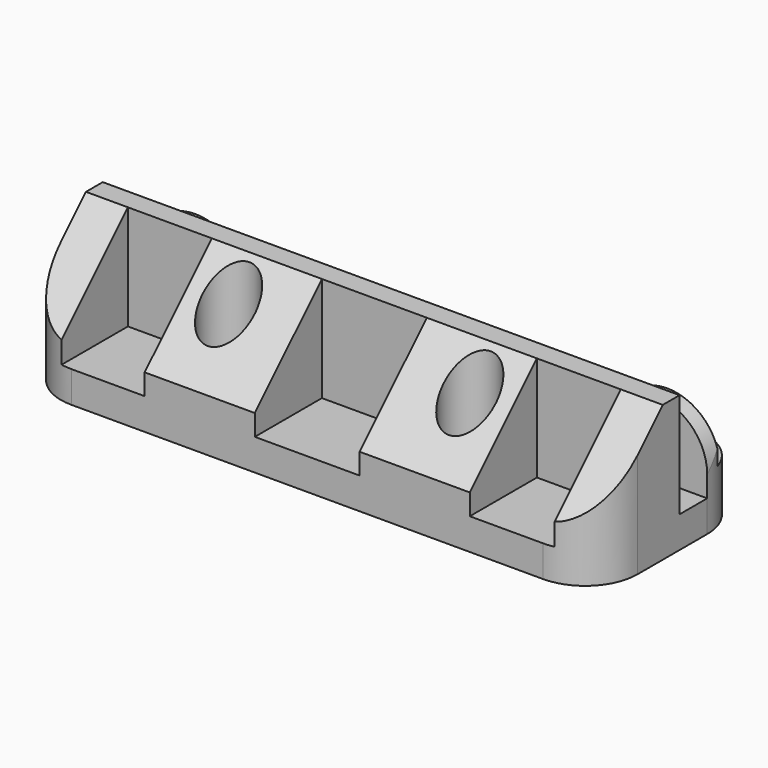
from build123d import *

# Parameters (mm, degrees)
F0_W         = 55
F0_H         = 18.3
F1_DEPTH     = 3
F2_W         = 55
F2_H         = 5
F3_DEPTH     = 2
F4_W         = 55
F4_H         = 10
F5_DEPTH     = 1
F6_W         = 10
F6_H         = 1.5
F7_DEPTH     = 5
F8_R         = 4.99999
F9_DEPTH     = 9
F11_R        = 1.6
F12_DEPTH    = 5
F13_R        = 1.6
F14_DEPTH    = 13
F15_W        = 10
F15_H        = 8
F15_W_2      = 8
F16_DEPTH    = 10
F17_R        = 2.5
F18_DEPTH    = 9
F19_T1_DEPTH = 45.1469278075
F19_T3_DEPTH = 51.6469278075
F19_T5_DEPTH = 51.6469278075
F19_T7_DEPTH = 45.1469278075
F20_T1_DEPTH = 30


# Not quite as in the source:
# - a fillet or chamfer that OpenCascade refuses, or shapes differently, is made with other operations: its cross-section is extruded or revolved along the edge and cut away or added
# - a fillet or chamfer is up to 0.001 mm smaller than in the source, because OpenCascade refuses the exact size


with BuildPart() as f1:
    # F0 (on Top) → F1 (new body)
    with BuildSketch(Plane.XY):
        Rectangle(F0_W, F0_H)
    extrude(amount=F1_DEPTH)

    # F2 (on face) → F3 (join)
    with BuildSketch(Plane.XY.offset(3)):
        with Locations((0, 6.65)):
            Rectangle(F2_W, F2_H)
    extrude(amount=F3_DEPTH)

    # F4 (on face) → F5 (join)
    with BuildSketch(Plane.XY.offset(3)):
        with Locations((0, -4.15)):
            Rectangle(F4_W, F4_H)
    extrude(amount=F5_DEPTH)

    # F6 (on face) → F7 (join)
    with BuildSketch(Plane.XY.offset(5)):
        with Locations((22.5, 4.9)):
            Rectangle(F6_W, F6_H)
        with Locations((-22.5, 4.9)):
            Rectangle(F6_W, F6_H)
    extrude(amount=F7_DEPTH)

    # F8 (radius 5 in the source; OpenCascade refuses exactly that, so slightly less here)
    f8_edges = [f1.edges().sort_by_distance(p)[0] for p in [
        (17.5, 4.9, 10),
        (27.5, 4.9, 10),
        (-27.5, 4.9, 10),
        (-17.5, 4.9, 10),
    ]]
    fillet(f8_edges, radius=F8_R)

    # F9 (add): a face of the model
    f9_faces = [f1.faces().sort_by_distance(p)[0] for p in [
        (0, -4.15, 4),
    ]]
    extrude(f9_faces, amount=F9_DEPTH)

    # F11 (on face) → F12 (cut)
    with BuildSketch(Plane.XY.offset(5)):
        with Locations((11.5, 6.65)):
            Circle(F11_R)
        with Locations((-11.5, 6.65)):
            Circle(F11_R)
    extrude(amount=-F12_DEPTH, mode=Mode.SUBTRACT)

    # F13 (on face) → F14 (cut)
    with BuildSketch(Plane.XY.offset(13)):
        with Locations((11.5, -4.15)):
            Circle(F13_R)
        with Locations((-11.5, -4.15)):
            Circle(F13_R)
    extrude(amount=-F14_DEPTH, mode=Mode.SUBTRACT)

    # F15 (on face) → F16 (cut)
    with BuildSketch(Plane.XY.offset(13)):
        with Locations((0, -5.15)):
            Rectangle(F15_W, F15_H)
        with Locations((19.5, -5.15)):
            Rectangle(F15_W_2, F15_H)
        with Locations((-19.5, -5.15)):
            Rectangle(F15_W_2, F15_H)
    extrude(amount=-F16_DEPTH, mode=Mode.SUBTRACT)

    # F17 (on face) → F18 (cut)
    with BuildSketch(Plane.XY.offset(13)):
        with Locations((11.5, -4.15)):
            Circle(F17_R)
        with Locations((-11.5, -4.15)):
            Circle(F17_R)
    extrude(amount=-F18_DEPTH, mode=Mode.SUBTRACT)

    # F19: chamfer of 8 on 4 edges, made by hand

    # F19_s2 → F19_t1 (cut)
    with BuildSketch(Plane.YZ.offset(2.9265360963)):
        Polygon((-1.15, 13), (-9.15, 5), (-9.15, 13), align=None)
    extrude(amount=F19_T1_DEPTH, mode=Mode.SUBTRACT)

    # F19_s4 → F19_t3 (cut)
    with BuildSketch(Plane.YZ.offset(-15.5734639037)):
        Polygon((-1.15, 13), (-9.15, 5), (-9.15, 13), align=None)
    extrude(amount=F19_T3_DEPTH, mode=Mode.SUBTRACT)

    # F19_s6 → F19_t5 (cut)
    with BuildSketch(Plane.YZ.offset(-36.0734639037)):
        Polygon((-1.15, 13), (-9.15, 5), (-9.15, 13), align=None)
    extrude(amount=F19_T5_DEPTH, mode=Mode.SUBTRACT)

    # F19_s8 → F19_t7 (cut)
    with BuildSketch(Plane.YZ.offset(-48.0734639037)):
        Polygon((-1.15, 13), (-9.15, 5), (-9.15, 13), align=None)
    extrude(amount=F19_T7_DEPTH, mode=Mode.SUBTRACT)

    # F20: fillet of radius 5 on 4 edges, made by hand

    # F20_s2 → F20_t1 (cut)
    with BuildSketch(Plane.XY.offset(-12.5)):
        with BuildLine():
            ThreePointArc((22.5, -9.15), (26.0355339059, -7.6855339059), (27.5, -4.15))
            Line((27.5, -4.15), (27.5, -9.15))
            Line((27.5, -9.15), (22.5, -9.15))
        make_face()
        with BuildLine():
            ThreePointArc((22.5, 9.15), (26.0355339059, 7.6855339059), (27.5, 4.15))
            Line((27.5, 4.15), (27.5, 9.15))
            Line((27.5, 9.15), (22.5, 9.15))
        make_face()
        with BuildLine():
            ThreePointArc((-22.5, 9.15), (-26.0355339059, 7.6855339059), (-27.5, 4.15))
            Line((-27.5, 4.15), (-27.5, 9.15))
            Line((-27.5, 9.15), (-22.5, 9.15))
        make_face()
        with BuildLine():
            ThreePointArc((-22.5, -9.15), (-26.0355339059, -7.6855339059), (-27.5, -4.15))
            Line((-27.5, -4.15), (-27.5, -9.15))
            Line((-27.5, -9.15), (-22.5, -9.15))
        make_face()
    extrude(amount=F20_T1_DEPTH, mode=Mode.SUBTRACT)


solid = f1.part
